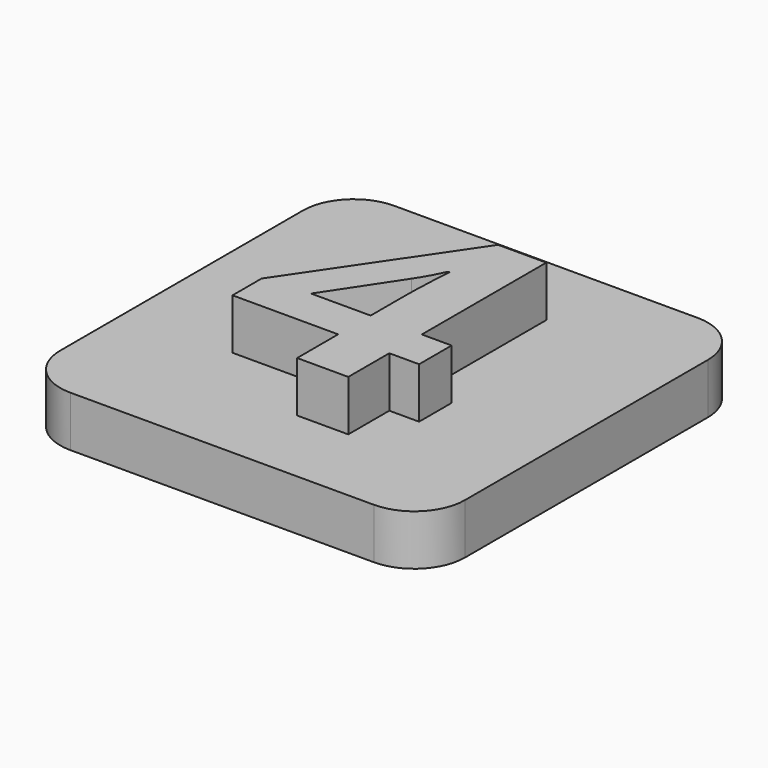
from build123d import *

# Parameters (mm, degrees)
F1_DEPTH     = 6.35
F2_TEXT_SIZE = 43.5149685169
F3_DEPTH     = 6.35


# Not quite as in the source:
# - Text() gives the source's letters only with a copy of the font that has no kerning and outlines rounded to 1/6400 em; it was checked with that copy


with BuildPart() as f1:
    # F0 (on Top) → F1 (new body)
    with BuildSketch(Plane.XY):
        with BuildLine():
            Line((-8.8098541204, 57.7911652245), (-46.9098541204, 57.7911652245))
            ThreePointArc((-46.9098541204, 57.7911652245), (-51.3999821809, 55.931293285), (-53.2598541204, 51.4411652245))
            Line((-53.2598541204, 51.4411652245), (-53.2598541204, 13.3411652245))
            ThreePointArc((-53.2598541204, 13.3411652245), (-51.3999821809, 8.8510371639), (-46.9098541204, 6.9911652245))
            Line((-46.9098541204, 6.9911652245), (-8.8098541204, 6.9911652245))
            ThreePointArc((-8.8098541204, 6.9911652245), (-4.3197260599, 8.8510371639), (-2.4598541204, 13.3411652245))
            Line((-2.4598541204, 13.3411652245), (-2.4598541204, 51.4411652245))
            ThreePointArc((-2.4598541204, 51.4411652245), (-4.3197260599, 55.931293285), (-8.8098541204, 57.7911652245))
        make_face()
    extrude(amount=F1_DEPTH)

    # F2 (on face) → F3 (join)
    with BuildSketch(Plane.XY.offset(6.35)):
        with Locations((-40.5228659511, 17.0895140618)):
            Text('4', F2_TEXT_SIZE, font='Open Sans', font_style=FontStyle.BOLD, text_align=(TextAlign.LEFT, TextAlign.BOTTOM))
    extrude(amount=F3_DEPTH)


solid = f1.part
